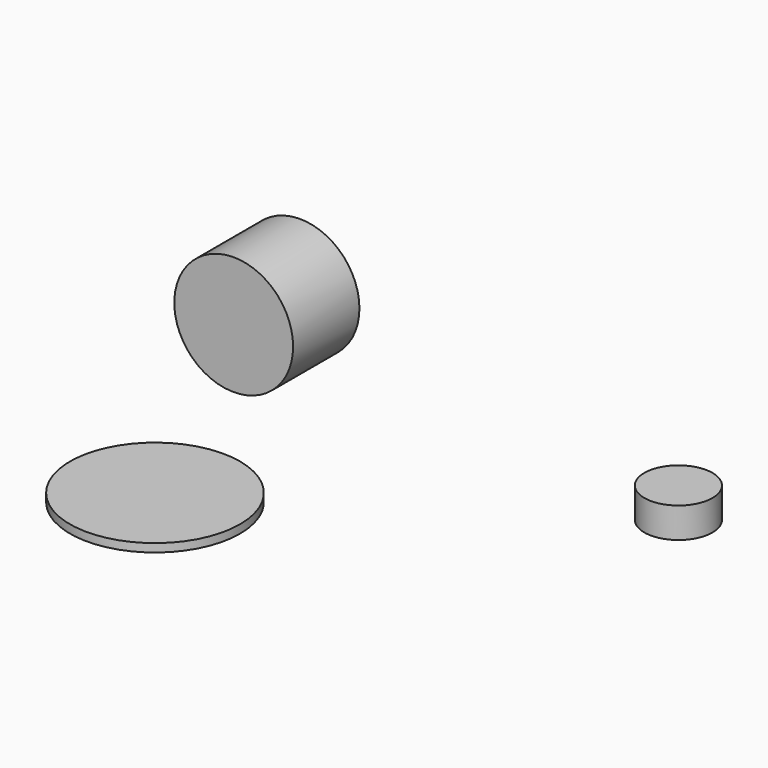
from build123d import *

# Parameters (mm, degrees)
F0_R     = 10.2656995883
F1_DEPTH = 9.1642085463
F2_R     = 25.6488599295
F3_DEPTH = 2.5
F4_R     = 17.9131946883
F5_DEPTH = 25


# Not quite as in the source:
# - the program builds the solid bodies; features that only make, move or delete a surface that nothing else refers to are left out


with BuildPart() as f1:
    # F0 (on Top) → F1 (new body)
    with BuildSketch(Plane.XY):
        with Locations((37.4742150307, 36.9413942099)):
            Circle(F0_R)
    extrude(amount=F1_DEPTH)


with BuildPart() as f3:
    # F2 (on Top) → F3 (new body)
    with BuildSketch(Plane.XY):
        with Locations((-64.4004046917, -33.0038070679)):
            Circle(F2_R)
    extrude(amount=F3_DEPTH)


with BuildPart() as f5:
    # F4 (on Front) → F5 (new body)
    with BuildSketch(Plane.XZ):
        with Locations((-47.0752343535, 49.5246499777)):
            Circle(F4_R)
    extrude(amount=F5_DEPTH)


solid = Compound([f1.part, f3.part, f5.part])
